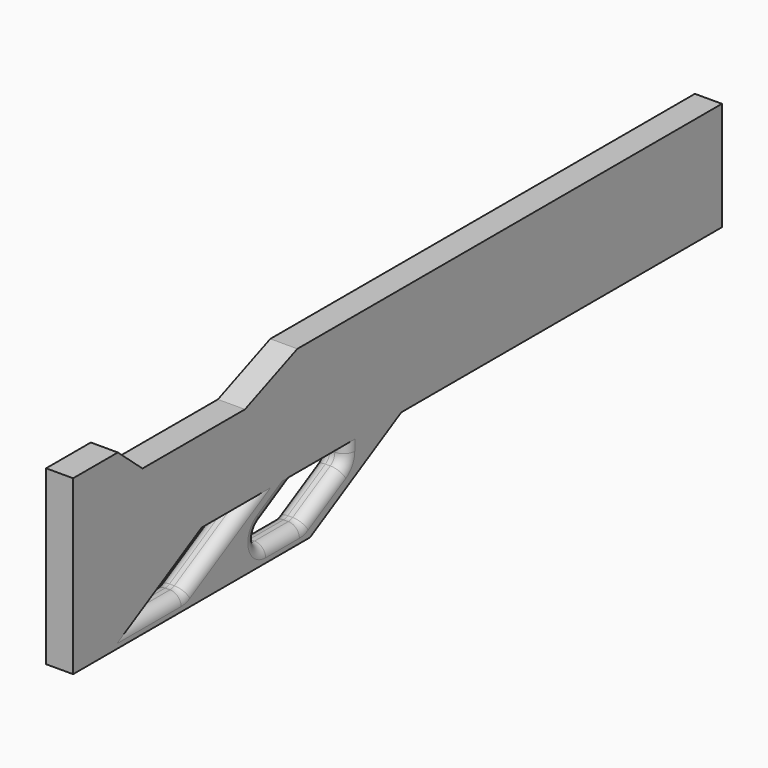
from build123d import *

# Parameters (mm, degrees)
F1_DEPTH = 10
F2_F1_R  = 8.2083261121
F2_F2_R  = 8.2083261121


with BuildPart() as f1:
    # F0 (on Right) → F1 (new body, symmetric)
    with BuildSketch(Plane.YZ):
        Polygon((-255.1260930291, 127.6137977839), (-296.4929085316, 127.6137977839), (-296.4929085316, 0), (-262.0377242565, 0), (-241.1511396352, 11.6772135656), (-177.6259690523, 47.1926890314), (-130.9504058889, 47.1926890314), (-86.4829342095, 47.1926890314), (-44.2343052483, 47.1926890314), (6.9967018189, 47.1926890314), (303.5070914684, 47.1926890314), (303.5070914684, 127.6137977839), (-89.1410559416, 127.6137977839), (-137.561365962, 107.9020351171), (-232.3477119207, 107.9020351171), align=None)
        Polygon((-241.1511396352, 11.6772135656), (-262.0377242565, 0), (-77.4150533853, 0), (6.9967018189, 47.1926890314), (-44.2343052483, 47.1926890314), (-44.2343052483, 34.5198116153), (-85.0919854182, 11.6772135656), (-150.0081047923, 11.6772135656), (-194.4755764717, 11.6772135656), align=None)
        Polygon((-130.9504058889, 47.1926890314), (-194.4755764717, 11.6772135656), (-150.0081047923, 11.6772135656), (-86.4829342095, 47.1926890314), align=None)
    extrude(amount=F1_DEPTH, both=True)

    # F2: fillet of radius 8.2083261121 on 12 edges, made by hand

    # F2_f1
    f2_f1_edges = [f1.edges().sort_by_distance(p)[0] for p in [
        (0, -150.0081047923, 11.6772135656),
        (0, -194.4755764717, 11.6772135656),
        (0, -85.0919854182, 11.6772135656),
        (0, -44.2343052483, 34.5198116153),
    ]]
    fillet(f2_f1_edges, radius=F2_F1_R)

    # F2_f2
    f2_f2_edges = [f1.edges().sort_by_distance(p)[0] for p in [
        (10, -161.7795821345, 29.9567990284),
        (-10, -161.7795821345, 29.9567990284),
        (-10, -104.4970100413, 37.1214296806),
        (10, -104.4970100413, 37.1214296806),
        (10, -126.4486219722, 17.8158787517),
        (-10, -126.4486219722, 17.8158787517),
        (-10, -194.5446792073, 11.9424218254),
        (10, -194.5446792073, 11.9424218254),
    ]]
    fillet(f2_f2_edges, radius=F2_F2_R)


solid = f1.part
